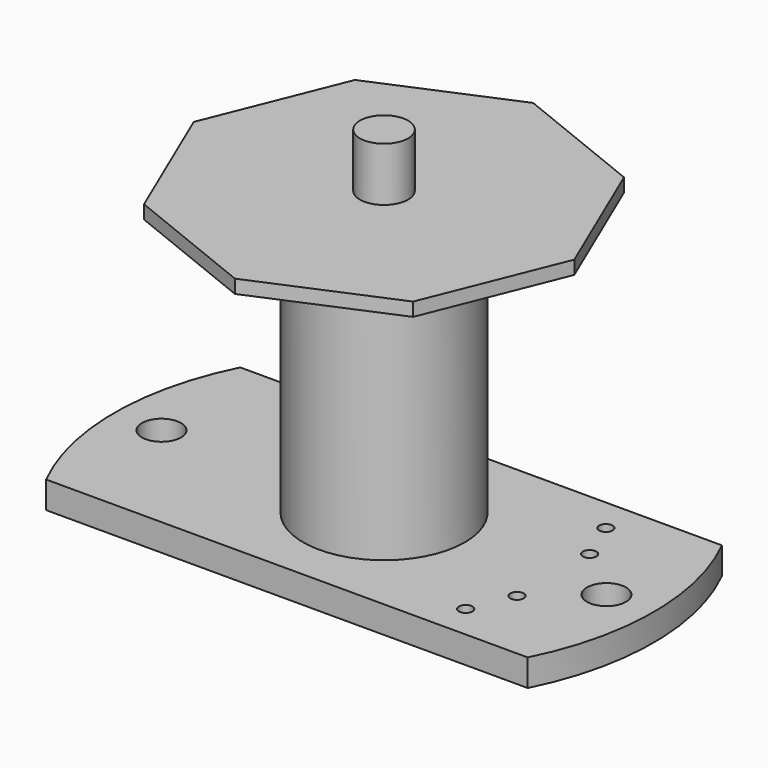
from build123d import *

# Parameters (mm, degrees)
F0_R      = 20
F0_R_2    = 1.45
F0_R_3    = 1.7859375
F1_DEPTH  = 2
F2_R      = 6
F2_R_2    = 1.7859375
F3_DEPTH  = 20
F4_R      = 1.7859375
F5_DEPTH  = 27
F6_R      = 1.7859375
F7_DEPTH  = 1
F9_DEPTH  = 25
F10_R     = 0.5
F11_DEPTH = 25


with BuildPart() as f1:
    # F0 (on Top) → F1 (new body)
    with BuildSketch(Plane.XY):
        Circle(F0_R)
        with Locations((-16.5, 0)):
            Circle(F0_R_2, mode=Mode.SUBTRACT)
        Circle(F0_R_3, mode=Mode.SUBTRACT)
        with Locations((16.5, 0)):
            Circle(F0_R_2, mode=Mode.SUBTRACT)
    extrude(amount=F1_DEPTH)

    # F8 (on face) → F9 (cut)
    with BuildSketch(Plane(origin=(0, 0, 0), x_dir=(1, 0, 0), z_dir=(0, 0, -1))):
        with BuildLine():
            ThreePointArc((17.8605710995, 9), (0, 20), (-17.8605710995, 9))
            Line((-17.8605710995, 9), (17.8605710995, 9))
        make_face()
        with BuildLine():
            Line((17.8605710995, -9), (-17.8605710995, -9))
            ThreePointArc((-17.8605710995, -9), (0, -20), (17.8605710995, -9))
        make_face()
    extrude(amount=-F9_DEPTH, mode=Mode.SUBTRACT)

    # F10 (on face) → F11 (cut)
    with BuildSketch(Plane(origin=(0, 0, 0), x_dir=(1, 0, 0), z_dir=(0, 0, -1))):
        with Locations((11.2583302492, 6.5)):
            Circle(F10_R)
        with Locations((12.5570357418, 3.3646475863)):
            Circle(F10_R)
        with Locations((12.5570357418, -3.3646475863)):
            Circle(F10_R)
        with Locations((11.2583302492, -6.5)):
            Circle(F10_R)
    extrude(amount=-F11_DEPTH, mode=Mode.SUBTRACT)


with BuildPart() as f3:
    # F2 (on face) → F3 (new body)
    with BuildSketch(Plane.XY.offset(2)):
        Circle(F2_R)
        Circle(F2_R_2, mode=Mode.SUBTRACT)
    extrude(amount=F3_DEPTH)


with BuildPart() as f5:
    # F4 (on face) → F5 (new body)
    with BuildSketch(Plane(origin=(0, 0, 0), x_dir=(1, 0, 0), z_dir=(0, 0, -1))):
        Circle(F4_R)
    extrude(amount=-F5_DEPTH)


with BuildPart() as f7:
    # F6 (on face) → F7 (new body)
    with BuildSketch(Plane.XY.offset(22)):
        Polygon((-0.1404503089, 13.9992954719), (-9.9983101259, 9.7996833942), (-13.9992954719, -0.1404503089), (-9.7996833942, -9.9983101259), (0.1404503089, -13.9992954719), (9.9983101259, -9.7996833942), (13.9992954719, 0.1404503089), (9.7996833942, 9.9983101259), align=None)
        Circle(F6_R, mode=Mode.SUBTRACT)
    extrude(amount=F7_DEPTH)


solid = Compound([f1.part, f3.part, f5.part, f7.part])
